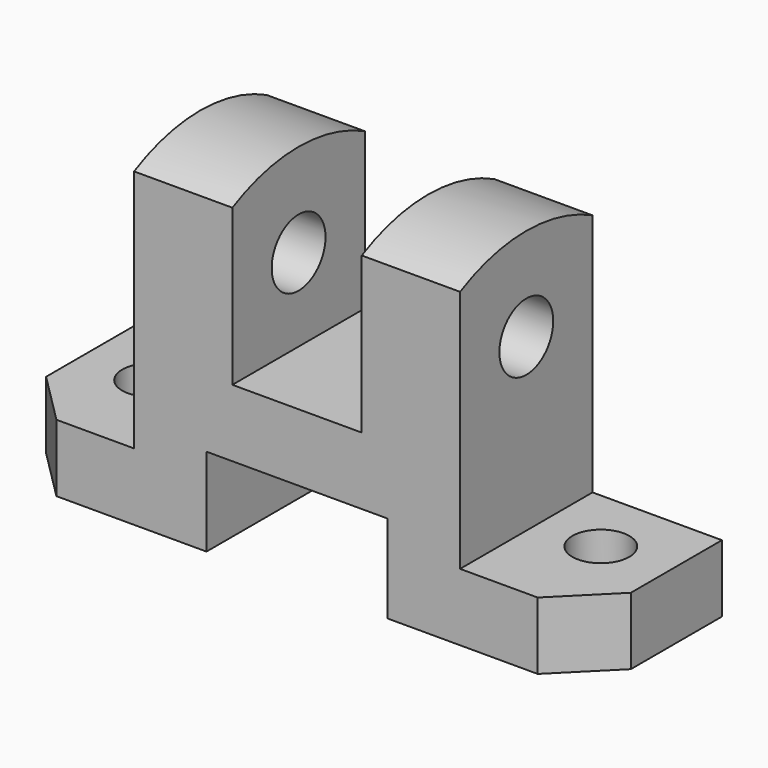
from build123d import *

# Parameters (mm, degrees)
F0_R     = 6.5
F1_DEPTH = 113
F2_W     = 25
F2_H     = 3.8712351675
F2_H_2   = 47.1287648325
F2_H_3   = 30.1287648325
F2_W_2   = 35
F2_H_4   = 17
F3_DEPTH = 32.001
F4_R     = 5.5
F5_DEPTH = 13.001


with BuildPart() as f1:
    # F0 (on Right) → F1 (new body)
    with BuildSketch(Plane.YZ):
        with BuildLine():
            Line((0, 60.1287648325), (0, 0))
            Line((0, 0), (32, 0))
            Line((32, 0), (32, 60.1287648325))
            ThreePointArc((32, 60.1287648325), (16, 64), (0, 60.1287648325))
        make_face()
        with Locations((16, 46)):
            Circle(F0_R, mode=Mode.SUBTRACT)
    extrude(amount=F1_DEPTH)

    # F2 (on face) → F3 (cut, through all)
    with BuildSketch(Plane.XZ):
        with Locations((12.5, 62.0643824163)):
            Rectangle(F2_W, F2_H)
        with Locations((12.5, 36.5643824163)):
            Rectangle(F2_W, F2_H_2)
        with Locations((56.5, 45.0643824163)):
            Rectangle(F2_W, F2_H_3)
        with Locations((56.5, 62.0643824163)):
            Rectangle(F2_W, F2_H)
        with Locations((100.5, 62.0643824163)):
            Rectangle(F2_W, F2_H)
        with Locations((100.5, 36.5643824163)):
            Rectangle(F2_W, F2_H_2)
        with Locations((56.5, 8.5)):
            Rectangle(F2_W_2, F2_H_4)
    extrude(amount=-F3_DEPTH, mode=Mode.SUBTRACT)

    # F4 (on face) → F5 (cut, through all)
    with BuildSketch(Plane.XY.offset(13)):
        Polygon((103, 0), (113, 0), (113, 10), align=None)
        with Locations((100, 19)):
            Circle(F4_R)
        with Locations((13, 19)):
            Circle(F4_R)
        Polygon((0, 10), (0, 0), (10, 0), align=None)
    extrude(amount=-F5_DEPTH, mode=Mode.SUBTRACT)


solid = f1.part
